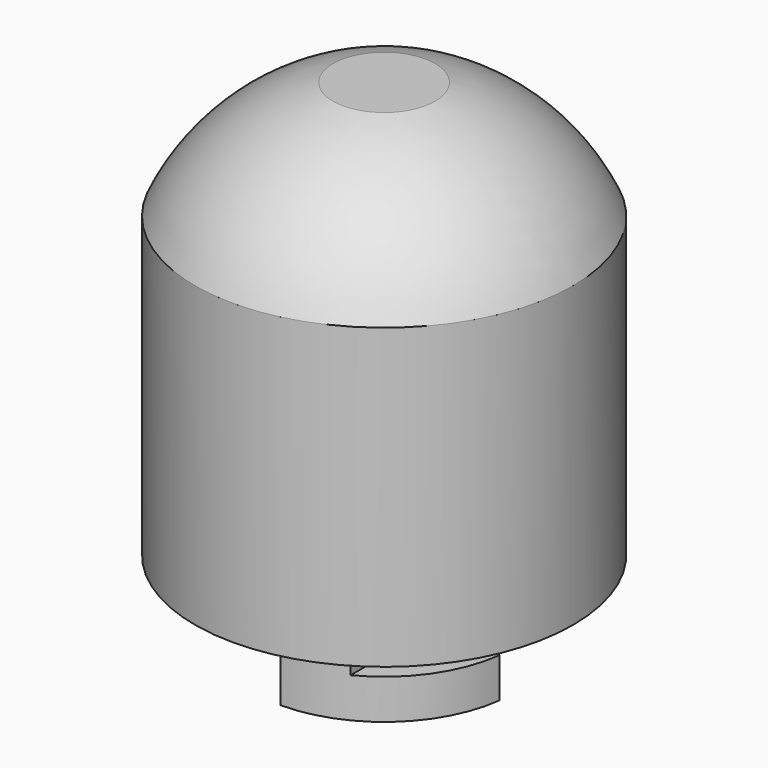
from build123d import *

# Parameters (mm, degrees)
F0_R     = 19
F0_R_2   = 17.5
F1_DEPTH = 30
F5_DEPTH = 2
F7_DEPTH = 8
F8_W     = 3.0304512245
F8_H     = 4
F8_W_2   = 3.9695487755
F9_DEPTH = 25


# Not quite as in the source:
# - a feature names something its author has since deleted; it is built from what else it names


with BuildPart() as f1:
    # F0 (on Top) → F1 (new body)
    with BuildSketch(Plane.XY):
        Circle(F0_R)
        Circle(F0_R_2, mode=Mode.SUBTRACT)
    extrude(amount=F1_DEPTH)

    # F2 (on Front) → F3 (revolve)
    with BuildSketch(Plane.XZ):
        with BuildLine():
            Line((0, 41.805047949), (0, 30))
            Line((0, 30), (19, 30))
            ThreePointArc((19, 30), (13.3813344534, 37.450646936), (5.1278058683, 41.805047949))
            Line((5.1278058683, 41.805047949), (0, 41.805047949))
        make_face()
    revolve(axis=Axis((0, 0, 35.9025239745), (0, 0, 1)))

    # F4 (on Top) → F5 (join)
    with BuildSketch(Plane.XY):
        with BuildLine():
            ThreePointArc((10, 0), (7.0710678119, -7.0710678119), (0, -10))
            Line((0, -10), (0, -19))
            ThreePointArc((0, -19), (13.4173031296, -13.4253390842), (18.972583327, 0))
            Line((18.972583327, 0), (10, 0))
        make_face()
    extrude(amount=F5_DEPTH)

    # F6 (on face) → F7 (join)
    with BuildSketch(Plane(origin=(0, 0, 0), x_dir=(1, 0, 0), z_dir=(0, 0, -1))):
        with BuildLine():
            Line((9.8692176419, 1.6119997323), (12.8996688664, 1.6119997323))
            ThreePointArc((12.8996688664, 1.6119997323), (8.6036039972, 9.745665614), (0, 13))
            Line((0, 13), (0, 10))
            ThreePointArc((0, 10), (6.4761100468, 7.6197111928), (9.8692176419, 1.6119997323))
        make_face()
    extrude(amount=F7_DEPTH)

    # F8 (on face) → F9 (cut)
    with BuildSketch(Plane(origin=(0, -1.6119997323, 0), x_dir=(-1, 0, 0), z_dir=(0, 1, 0))):
        with Locations((-11.3844432541, -2)):
            Rectangle(F8_W, F8_H)
        with Locations((-7.8844432541, -2)):
            Rectangle(F8_W_2, F8_H)
    extrude(amount=-F9_DEPTH, mode=Mode.SUBTRACT)


solid = f1.part
